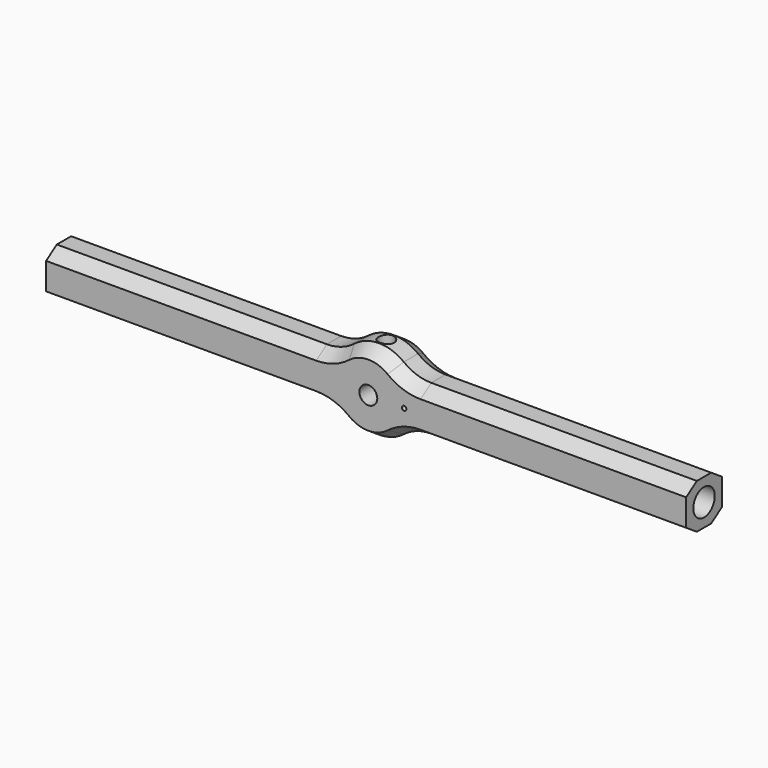
from build123d import *

# Parameters (mm, degrees)
F0_R          = 2
F0_R_2        = 0.5
F1_DEPTH      = 10
F2_R          = 3
F3_DEPTH      = 40
F4_R          = 1.75
F5_DEPTH      = 9.001
F5_DEPTH_BACK = 9.001
F6_R          = 10
F7_SIZE2      = 3
F7_SIZE       = 2
F7_2_SIZE2    = 3
F7_2_SIZE     = 2


# Not quite as in the source:
# - a pattern or mirror of a feature is missing from the dataset's text; its kind, count and spacing are read off the source's solid


with BuildPart() as f1:
    # F0 (on Front) → F1 (new body)
    with BuildSketch(Plane.XZ):
        with BuildLine():
            Line((71, 5), (7.4833147735, 5))
            ThreePointArc((7.4833147735, 5), (0, 9), (-7.4833147735, 5))
            Line((-7.4833147735, 5), (-72, 5))
            Line((-72, 5), (-72, -5))
            Line((-72, -5), (-7.4833147735, -5))
            ThreePointArc((-7.4833147735, -5), (0, -9), (7.4833147735, -5))
            Line((7.4833147735, -5), (71, -5))
            Line((71, -5), (71, 5))
        make_face()
        Circle(F0_R, mode=Mode.SUBTRACT)
        with Locations((8, 0)):
            Circle(F0_R_2, mode=Mode.SUBTRACT)
    extrude(amount=F1_DEPTH)

    # F2 (on face) → F3 (cut)
    with BuildSketch(Plane(origin=(-72, 0, 0), x_dir=(0, -1, 0), z_dir=(-1, 0, 0))):
        with Locations((5, 0)):
            Circle(F2_R)
    f3 = extrude(amount=-F3_DEPTH, mode=Mode.SUBTRACT)

    # F3_copies: F3 across plane
    add(f3.mirror(Plane(origin=(0, 0, 0), x_dir=(0, 0, 1), z_dir=(1, 0, 0))), mode=Mode.SUBTRACT)

    # F4 (on Top) → F5 (cut, two sides)
    with BuildSketch(Plane.XY) as f5_sk:
        with Locations((0, -5)):
            Circle(F4_R)
    extrude(amount=-F5_DEPTH, mode=Mode.SUBTRACT)
    extrude(f5_sk.sketch, amount=F5_DEPTH_BACK, mode=Mode.SUBTRACT)

    # F6
    f6_edges = [f1.edges().sort_by_distance(p)[0] for p in [
        (-7.483315, -5, 5),
        (7.483315, -5, 5),
        (7.483315, -5, -5),
        (-7.483315, -5, -5),
    ]]
    fillet(f6_edges, radius=F6_R)

    # F7
    f7_edges = [f1.edges().sort_by_distance(p)[0] for p in [
        (-41.830952, -10, 5),
        (-41.830952, -10, -5),
    ]]
    f7_side = f1.faces().sort_by_distance((41.330952, -10, -3.558716))[0]
    chamfer(f7_edges, length=F7_SIZE, length2=F7_SIZE2, reference=f7_side)

    # F7#2
    f7_2_edges = [f1.edges().sort_by_distance(p)[0] for p in [
        (-41.830952, 0, 5),
        (-41.830952, 0, -5),
    ]]
    f7_2_side = f1.faces().sort_by_distance((41.330952, 0, -3.558716))[0]
    chamfer(f7_2_edges, length=F7_2_SIZE, length2=F7_2_SIZE2, reference=f7_2_side)


solid = f1.part
